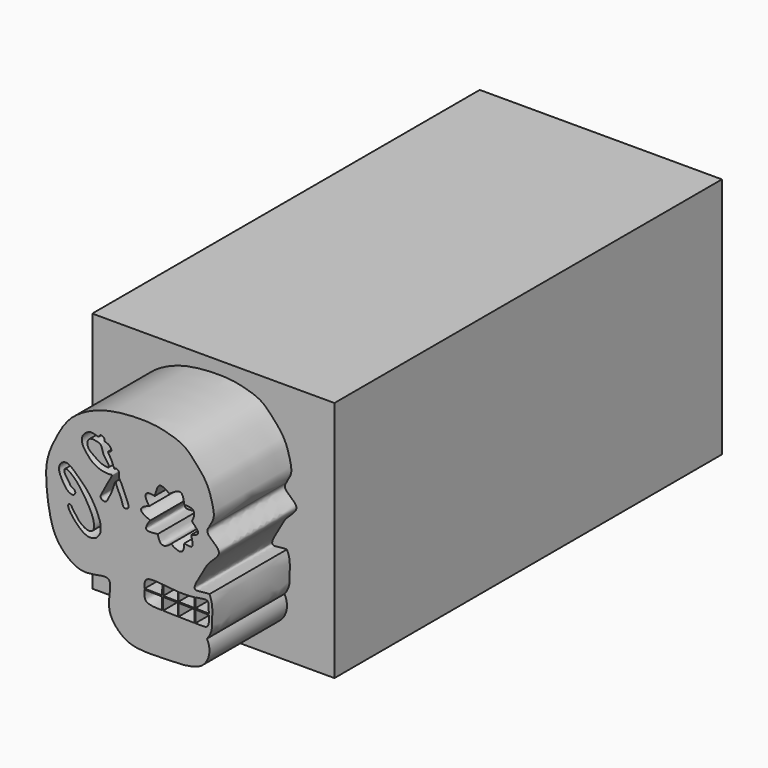
from build123d import *

# Parameters (mm, degrees)
F2_DEPTH = 5.08
F4_DEPTH = 2.54
F1_W     = 12.7
F1_H     = 12.7
F5_DEPTH = 25.4
F7_DEPTH = 2.54


# Not quite as in the source:
# - a feature names something its author has since deleted; it is built from what else it names


with BuildPart() as f2:
    # F0 (on Front) → F2 (new body)
    with BuildSketch(Plane.XZ):
        with BuildLine():
            add(Edge.make_bspline(
                [(-4.5544075169, 1.3928102558), (-3.9892874978, 1.3936850005), (-3.4668862346, 1.4183520112), (-2.9626822173, 1.6524156046)],
                knots=[0, 0, 0, 0, 1.6127567598, 1.6127567598, 1.6127567598, 1.6127567598], degree=3))
            ThreePointArc((-2.9626822173, 1.6524156046), (-2.5207832675, 2.2763871387), (-2.6206157382, 3.0344429644))
            add(Edge.make_bspline(
                [(-2.4891644716, 5.1324297674), (-2.3917935509, 4.9163684072), (-2.3253208599, 4.6052474923), (-2.353390935, 4.1438424987), (-2.3281786078, 3.742489633), (-2.3932487238, 3.3100298606), (-2.6206157382, 3.0344429644)],
                knots=[0, 0, 0, 0, 0.2589698298, 0.4843279934, 0.6967977434, 1, 1, 1, 1], degree=3))
            add(Edge.make_bspline(
                [(-2.4891644716, 5.1324297674), (-2.8544493428, 5.1336356945), (-3.5672375297, 4.8785009618), (-2.8152049208, 6.0650838014), (-2.5884297024, 6.5663222822), (-1.7654979463, 7.1854603195), (-2.3447073669, 7.6364237388), (-2.7154974719, 7.9931282788), (-2.5049047545, 8.2173803821)],
                knots=[0, 0, 0, 0, 0.1716411, 0.3609103093, 0.5270907012, 0.6999372879, 0.8498725142, 1, 1, 1, 1], degree=3))
            add(Edge.make_bspline(
                [(-8.4889251739, 4.0800906718), (-8.7589659452, 4.0356777743), (-9.3664055338, 3.9357737781), (-10.5025798395, 4.8392058498), (-10.9059573733, 6.1149046303), (-11.0740084695, 7.5770614576), (-11.0572913783, 8.6481895291), (-10.5066556684, 9.8561725352), (-9.801754858, 11.0173560965), (-8.5112279732, 11.7040800215), (-7.5130409963, 11.949362548), (-6.5368197907, 12.0472622026), (-5.4793488606, 12.0464613388), (-4.709549558, 11.8804829441), (-3.8077392578, 11.6081842347), (-3.2731241454, 11.0134554774), (-2.6219451437, 10.30229784), (-2.3610549942, 9.4868714168), (-2.171059183, 8.6611482213), (-2.4550122068, 8.385969167), (-2.5049047545, 8.2173803821)],
                knots=[0, 0, 0, 0, 0.0500780332, 0.1130041956, 0.1768956978, 0.2430992912, 0.299601719, 0.3619066714, 0.4259636055, 0.4912026128, 0.546777757, 0.6011196121, 0.6571512931, 0.7063637819, 0.7583810191, 0.807340639, 0.8606442381, 0.9121796378, 0.9605447696, 1, 1, 1, 1], degree=3))
            add(Edge.make_bspline(
                [(-8.4889251739, 4.0800906718), (-8.1891140401, 4.1435086925), (-7.5824093701, 4.2718428501), (-7.7738611768, 3.2641836277), (-7.7788952185, 2.4127249564), (-6.96730618, 1.53934763), (-6.0435092719, 1.3353211789), (-5.0895326997, 1.3721509203), (-4.5544075169, 1.3928102558)],
                knots=[0, 0, 0, 0, 0.1444018704, 0.2922149289, 0.4524717395, 0.6284063598, 0.7915576541, 1, 1, 1, 1], degree=3))
        make_face()
    extrude(amount=F2_DEPTH)

    # F3 (on face) → F4 (cut)
    with BuildSketch(Plane.XZ.offset(5.08)):
        with BuildLine():
            add(Edge.make_bspline(
                [(-5.3659848497, 8.7208530881), (-5.2846155708, 8.9727846377), (-5.1710596458, 9.5011555318), (-4.7726393834, 9.210328647), (-4.5891036161, 9.0864328929)],
                knots=[0, 0, 0, 0, 0.5208455257, 1, 1, 1, 1], degree=3))
            add(Edge.make_bspline(
                [(-5.6486829395, 8.1671502605), (-5.8447078545, 8.4470894225), (-5.89391753, 8.7083353104), (-5.6496376746, 8.8005099615), (-5.3659848497, 8.7208530881)],
                knots=[0, 0, 0, 0, 0.5203515764, 1, 1, 1, 1], degree=3))
            add(Edge.make_bspline(
                [(-5.5914319294, 7.523380365), (-5.9265031703, 7.6624876681), (-6.211049844, 7.8478040514), (-5.9524201806, 8.0796377028), (-5.6486829395, 8.1671502605)],
                knots=[0, 0, 0, 0, 0.5158761073, 1, 1, 1, 1], degree=3))
            add(Edge.make_bspline(
                [(-5.205368324, 7.020722894), (-5.515797094, 6.9918642839), (-5.9481758185, 6.9293833828), (-5.7582442305, 7.3223857959), (-5.5914319294, 7.523380365)],
                knots=[0, 0, 0, 0, 0.5169308821, 1, 1, 1, 1], degree=3))
            add(Edge.make_bspline(
                [(-4.503384329, 6.7972433223), (-4.6912512029, 6.6368405751), (-5.0149208939, 6.4855239947), (-5.1457634756, 6.7906186317), (-5.205368324, 7.020722894)],
                knots=[0, 0, 0, 0, 0.5060867221, 1, 1, 1, 1], degree=3))
            add(Edge.make_bspline(
                [(-3.8085296017, 7.0489807986), (-3.8179540305, 6.8205589246), (-3.9035421605, 6.4800894964), (-4.2735109706, 6.6416122857), (-4.503384329, 6.7972433223)],
                knots=[0, 0, 0, 0, 0.4741735792, 1, 1, 1, 1], degree=3))
            add(Edge.make_bspline(
                [(-3.4450484308, 7.5613067453), (-3.3931593436, 7.3388874407), (-3.2822488519, 6.9007696507), (-3.643370237, 7.0191586974), (-3.8085296017, 7.0489807986)],
                knots=[0, 0, 0, 0, 0.5361984101, 1, 1, 1, 1], degree=3))
            add(Edge.make_bspline(
                [(-3.4099325727, 8.2039631478), (-3.2352017889, 8.026130414), (-2.9070428182, 7.6933064131), (-3.2817976238, 7.6055767004), (-3.4450484308, 7.5613067453)],
                knots=[0, 0, 0, 0, 0.544051219, 1, 1, 1, 1], degree=3))
            add(Edge.make_bspline(
                [(-3.8085296017, 8.8362629435), (-3.5648082767, 8.8254965564), (-3.2197177366, 8.7894369685), (-3.2957520719, 8.4058710656), (-3.4099325727, 8.2039631478)],
                knots=[0, 0, 0, 0, 0.498752658, 1, 1, 1, 1], degree=3))
            add(Edge.make_bspline(
                [(-4.5891036161, 9.0864328929), (-4.3604972194, 9.2348500345), (-3.9239269227, 9.5411548249), (-3.8456756119, 9.0618850519), (-3.8085296017, 8.8362629435)],
                knots=[0, 0, 0, 0, 0.5208679793, 1, 1, 1, 1], degree=3))
        make_face()
        with BuildLine():
            add(Edge.make_bspline(
                [(-2.5100025301, 4.2244921883), (-2.520578067, 4.3152952205), (-2.5578180106, 4.4604788228), (-2.5158321387, 4.7109072782), (-2.5786668798, 4.7712087792)],
                knots=[0.897450569, 0.897450569, 0.897450569, 0.897450569, 0.943851131, 1, 1, 1, 1], degree=3))
            add(Edge.make_bspline(
                [(-2.5786668798, 4.7712087792), (-2.6704912661, 4.8593311814), (-2.9455983215, 4.7834076397), (-3.2307982195, 4.740927492)],
                knots=[0, 0, 0, 0, 0.082053898, 0.082053898, 0.082053898, 0.082053898], degree=3))
            Line((-3.2307982195, 4.740927492), (-3.2307982195, 4.2372223453))
            Line((-3.2307982195, 4.2372223453), (-2.5100025301, 4.2244921883))
        make_face()
        with BuildLine():
            Line((-3.2835614095, 4.2381542095), (-3.2835614095, 4.733464152))
            add(Edge.make_bspline(
                [(-3.2835614095, 4.733464152), (-3.5464724783, 4.6982316498), (-3.818837814, 4.6907418319), (-4.1149102539, 4.7047607206)],
                knots=[0.087102599, 0.087102599, 0.087102599, 0.087102599, 0.1623975177, 0.1623975177, 0.1623975177, 0.1623975177], degree=3))
            Line((-4.1149102539, 4.7047607206), (-4.1149102539, 4.252836874))
            Line((-4.1149102539, 4.252836874), (-3.2835614095, 4.2381542095))
        make_face()
        with BuildLine():
            add(Edge.make_bspline(
                [(-3.2307982195, 3.5453085469), (-3.0819196309, 3.5437212449), (-2.7845176535, 3.5423901635), (-2.5236034229, 3.5540879015), (-2.4932600243, 3.9950860378), (-2.5042828638, 4.1620978154)],
                knots=[0.7162270597, 0.7162270597, 0.7162270597, 0.7162270597, 0.7598282834, 0.8127851111, 0.8874922891, 0.8874922891, 0.8874922891, 0.8874922891], degree=3))
            Line((-2.5042828638, 4.1620978154), (-3.2307982195, 4.1771585824))
            Line((-3.2307982195, 4.1771585824), (-3.2307982195, 3.5453085469))
        make_face()
        with BuildLine():
            Line((-4.1466693964, 4.2533977804), (-4.1466693964, 4.7063419309))
            add(Edge.make_bspline(
                [(-4.1466693964, 4.7063419309), (-4.2841026724, 4.7135161864), (-4.5281383074, 4.7335543048), (-4.7913856842, 4.7650778716), (-4.8995402052, 4.7771011772)],
                knots=[0.1650820479, 0.1650820479, 0.1650820479, 0.1650820479, 0.199832505, 0.2245551922, 0.2245551922, 0.2245551922, 0.2245551922], degree=3))
            Line((-4.8995402052, 4.7771011772), (-4.9101171375, 4.2668812262))
            Line((-4.9101171375, 4.2668812262), (-4.1466693964, 4.2533977804))
        make_face()
        with BuildLine():
            Line((-3.2835614095, 3.5459043926), (-3.2835614095, 4.1782523708))
            Line((-3.2835614095, 4.1782523708), (-4.1149102539, 4.1954863509))
            Line((-4.1149102539, 4.1954863509), (-4.1149102539, 3.5604707833))
            add(Edge.make_bspline(
                [(-4.1149102539, 3.5604707833), (-4.0408241734, 3.5589141905), (-3.7698923023, 3.553373967), (-3.4757319857, 3.5481906988), (-3.2835614095, 3.5459043926)],
                knots=[0.6348464492, 0.6348464492, 0.6348464492, 0.6348464492, 0.6560325596, 0.7111320672, 0.7111320672, 0.7111320672, 0.7111320672], degree=3))
        make_face()
        with BuildLine():
            Line((-4.9716904084, 4.2679686874), (-4.9609968604, 4.7838140535))
            add(Edge.make_bspline(
                [(-4.9609968604, 4.7838140535), (-5.3208727003, 4.8223180899), (-5.9235275829, 4.8579731181), (-5.8932860938, 4.4631796385), (-5.8910857477, 4.2842063637)],
                knots=[0.2292508395, 0.2292508395, 0.2292508395, 0.2292508395, 0.3120114738, 0.3777827863, 0.3777827863, 0.3777827863, 0.3777827863], degree=3))
            Line((-5.8910857477, 4.2842063637), (-4.9716904084, 4.2679686874))
        make_face()
        with BuildLine():
            Line((-4.1466693964, 3.5611405954), (-4.1466693964, 4.1961447225))
            Line((-4.1466693964, 4.1961447225), (-4.9112549433, 4.2119946899))
            Line((-4.9112549433, 4.2119946899), (-4.9243966083, 3.5780547668))
            add(Edge.make_bspline(
                [(-4.9243966083, 3.5780547668), (-4.6595247666, 3.5724955244), (-4.4098866766, 3.5667124744), (-4.1466693964, 3.5611405954)],
                knots=[0.5562162986, 0.5562162986, 0.5562162986, 0.5562162986, 0.631812493, 0.631812493, 0.631812493, 0.631812493], degree=3))
        make_face()
        with BuildLine():
            Line((-4.9728242986, 4.2132710314), (-5.8908832805, 4.2323025251))
            add(Edge.make_bspline(
                [(-5.8908832805, 4.2323025251), (-5.8908855296, 4.2319734461), (-5.8922755687, 4.035750978), (-5.9627191929, 3.5977162792), (-5.3308504169, 3.5864270768), (-5.0023696566, 3.5796748174)],
                knots=[0.3841354869, 0.3841354869, 0.3841354869, 0.3841354869, 0.3842563844, 0.4562266493, 0.5488422034, 0.5488422034, 0.5488422034, 0.5488422034], degree=3))
            add(Edge.make_bspline(
                [(-5.0023696566, 3.5796748174), (-4.996894276, 3.5795622654), (-4.9914264206, 3.5794496023), (-4.985965845, 3.5793368318)],
                knots=[0.5488422034, 0.5488422034, 0.5488422034, 0.5488422034, 0.5503859937, 0.5503859937, 0.5503859937, 0.5503859937], degree=3))
            Line((-4.985965845, 3.5793368318), (-4.9728242986, 4.2132710314))
        make_face()
    extrude(amount=-F4_DEPTH, mode=Mode.SUBTRACT)

    # F1 (on Front) → F5 (join)
    with BuildSketch(Plane.XZ):
        with Locations((-6.35, 6.35)):
            Rectangle(F1_W, F1_H)
    extrude(amount=-F5_DEPTH)

    # F6 (on face) → F7 (cut)
    with BuildSketch(Plane.XZ.offset(5.08)):
        with BuildLine():
            add(Edge.make_bspline(
                [(-7.7940328047, 9.9933389574), (-7.8218177192, 9.9521668322), (-7.6622061528, 9.7407230904), (-7.5832987765, 9.5394167034), (-7.4610042765, 9.2234030035), (-7.425314159, 9.3739783149), (-7.2956858026, 9.3085490242), (-7.1915929129, 9.1943703988), (-7.279465236, 8.9869246815), (-7.1078185466, 8.7765500756), (-6.91102714, 8.2761130639), (-6.7527025888, 7.9298549284), (-6.7088013625, 7.7316687619), (-6.8350132012, 7.650475367), (-7.0312750971, 7.6472982023), (-7.0724224471, 8.0378407766), (-7.3894831717, 8.5386162625), (-7.4079891278, 8.806522289), (-7.5306681281, 8.4268637268), (-7.6273648912, 8.1332841601), (-7.7951582028, 7.8318099119), (-7.8723857954, 7.6475014251), (-8.0588882827, 7.5974009486), (-8.2593199551, 7.765359758), (-8.0729417121, 8.0235503776), (-7.9266339536, 8.4027448375), (-7.510657191, 9.0237207446), (-7.7391716253, 8.9435121654), (-7.9853512843, 8.9823328733), (-8.2427354579, 9.0115569707), (-8.5896382909, 9.1870153579), (-8.8254060311, 9.4126056092), (-9.0589504097, 9.7049687495), (-9.1787740034, 9.924279229), (-9.2018891863, 10.2965849178), (-8.8699280325, 10.5618649917), (-8.6339260227, 10.6183040642), (-8.2628645677, 10.4474503291), (-8.2338067546, 10.6565790042), (-8.0744503854, 10.5804944066), (-7.9726672524, 10.5176288242), (-8.0196798787, 10.3860556136), (-7.8160551181, 10.3591032399), (-7.6583686503, 10.2277446923), (-7.5994807555, 10.0163628558), (-7.7721156719, 10.0258161109), (-7.7940328047, 9.9933389574)],
                knots=[0, 0, 0, 0, 0.0230209194, 0.048198217, 0.0706796709, 0.0825155829, 0.0981348752, 0.1157016104, 0.1356071624, 0.1587911135, 0.1931441993, 0.2223450708, 0.2413324319, 0.2577350726, 0.2752571451, 0.3026337457, 0.3397892089, 0.356629672, 0.3807034579, 0.4086867869, 0.43555553, 0.455632199, 0.4742940452, 0.4947569502, 0.5179859583, 0.5506491169, 0.5860249376, 0.6012950047, 0.6248998256, 0.6486979268, 0.6770200654, 0.7039260903, 0.7318320091, 0.7550160082, 0.7818181659, 0.8105321463, 0.8338884817, 0.8605474649, 0.8765138688, 0.8937131412, 0.9092473419, 0.9233226221, 0.9421191312, 0.963817332, 0.9818407739, 1, 1, 1, 1], degree=3))
        make_face()
        with BuildLine():
            add(Edge.make_bspline(
                [(-8.1962291151, 10.1776784286), (-8.1376326351, 10.1127513881), (-8.1008190947, 9.8667666188), (-7.9451032422, 9.5924853502), (-7.6092167699, 9.1905107024), (-8.2281827147, 9.3025046699), (-8.5090627034, 9.5520615973), (-8.8790158012, 9.755764026), (-8.9236779075, 10.1424698141), (-8.7047279976, 10.3274133734), (-8.4249155173, 10.2697102456), (-8.2486703499, 10.2357852325), (-8.1962291151, 10.1776784286)],
                knots=[0, 0, 0, 0, 0.096362847, 0.2026621177, 0.3017274166, 0.4126826773, 0.5274399391, 0.6367761518, 0.736927785, 0.8219240544, 0.9137595521, 1, 1, 1, 1], degree=3))
        make_face(mode=Mode.SUBTRACT)
        with BuildLine():
            add(Edge.make_bspline(
                [(-9.545262903, 7.6136770658), (-9.5142695388, 7.5652628949), (-9.5307035345, 7.423307781), (-9.6987162158, 7.3585660506), (-9.9876688425, 7.4957016444), (-10.2189171225, 7.8971406879), (-10.4225719444, 8.2906388098), (-10.3263962107, 8.6641792982), (-10.0184495652, 8.8014967626), (-9.7731848415, 8.6857402005), (-9.4857824297, 8.4285358514), (-9.1390493006, 8.1043496751), (-8.7456855022, 7.6810368428), (-8.4028632746, 7.094209414), (-8.3026793355, 6.8106503423), (-8.1689936228, 6.4751429165), (-8.2071063611, 6.2121524584), (-8.1718544304, 6.1397869475), (-8.3784670203, 5.796783529), (-8.5344178296, 5.7439515937), (-8.7676710908, 5.6872020245), (-9.0768310344, 5.784943662), (-9.4103288174, 6.0646363795), (-9.6625429325, 6.350198517), (-9.9528622837, 6.7543398748), (-9.8496142543, 6.9434219779), (-9.7283504591, 6.8696786187), (-9.6613075047, 6.7161928409), (-9.4936015169, 6.5264499572), (-9.3743112017, 6.3117986514), (-9.1451529258, 6.1328087569), (-8.8998538671, 5.987237372), (-8.5785225221, 6.0075191908), (-8.5058290592, 6.4276996493), (-8.7287257144, 7.0291157723), (-9.127393792, 7.6468839665), (-9.4409882238, 8.0789121081), (-9.7865599714, 8.3852952368), (-9.9600300925, 8.4800134361), (-10.0782471273, 8.4667658038), (-10.1163056547, 8.339267713), (-10.0303079767, 8.139168805), (-9.8408205963, 7.895473211), (-9.7474491345, 7.713269466), (-9.5800579177, 7.6680297261), (-9.545262903, 7.6136770658)],
                knots=[0, 0, 0, 0, 0.0174376906, 0.0337223409, 0.0565901135, 0.0857600488, 0.1140094319, 0.1388148294, 0.1616826101, 0.182930536, 0.209202083, 0.2385149438, 0.2714855051, 0.3062090721, 0.3298381646, 0.355307561, 0.3762922269, 0.387982502, 0.4137028629, 0.4313853731, 0.4513715625, 0.475279677, 0.5030004414, 0.5304382085, 0.5595848806, 0.5754389391, 0.5889843217, 0.60651904, 0.6278624488, 0.6489952549, 0.6717366553, 0.6946044611, 0.7160945458, 0.7411161494, 0.7754860094, 0.8122142189, 0.8437766815, 0.8723626416, 0.8907892537, 0.9038188506, 0.9176778239, 0.9374063431, 0.9612509379, 0.9804233997, 1, 1, 1, 1], degree=3))
        make_face()
    extrude(amount=-F7_DEPTH, mode=Mode.SUBTRACT)


solid = f2.part
